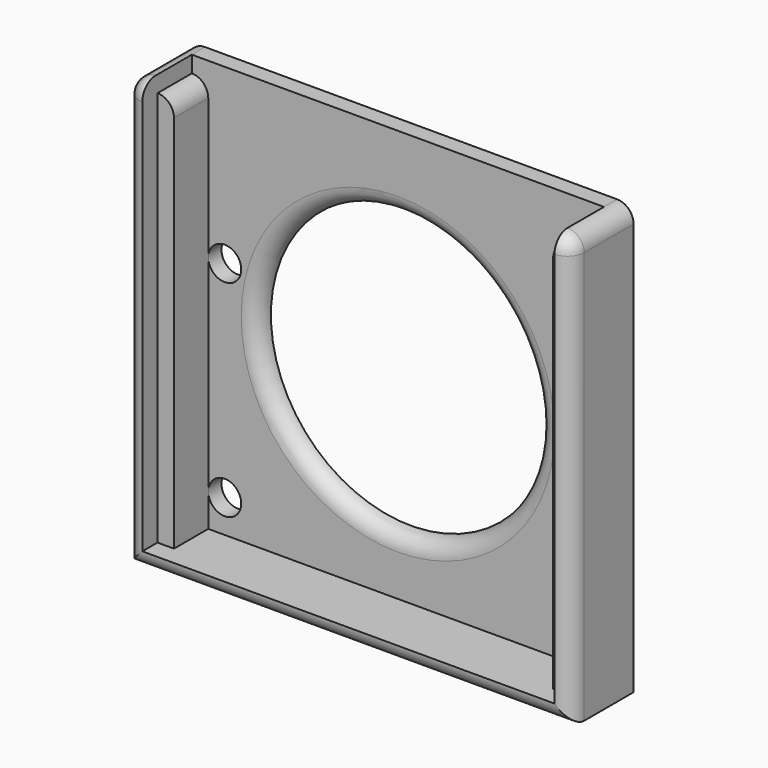
from build123d import *

# Parameters (mm, degrees)
F0_W     = 23
F0_H     = 1
F0_W_2   = 1
F1_DEPTH = 3.75
F2_DEPTH = 2.6
F0_R     = 1
F0_R_2   = 8.5
F3_DEPTH = 1
F4_R     = 0.99999


# Not quite as in the source:
# - a fillet or chamfer is up to 0.001 mm smaller than in the source, because OpenCascade refuses the exact size


with BuildPart() as f1:
    # F0 (on Front) → F1 (new body)
    with BuildSketch(Plane.XZ):
        Polygon((-12.5, -13), (-12.5, -12), (-12.5, 12), (-12.5, 13), (-13.5, 13), (-13.5, -13), align=None)
        Polygon((12.5, 12), (12.5, -12), (12.5, -13), (13.5, -13), (13.5, 13), (12.5, 13), align=None)
        with Locations((0, -12.5)):
            Rectangle(F0_W, F0_H)
        with Locations((-12, -12.5)):
            Rectangle(F0_W_2, F0_H)
        with Locations((12, -12.5)):
            Rectangle(F0_W_2, F0_H)
    extrude(amount=F1_DEPTH)

    # F0 (on Front) → F2 (join)
    with BuildSketch(Plane.XZ):
        Polygon((-12.5, -12), (-11.5, -12), (-11.5, -10), (-11.5, 2.5), (-11.5, 12), (-12.5, 12), align=None)
        Polygon((11.5, -12), (12.5, -12), (12.5, 12), (11.5, 12), (11.5, 2.5), (11.5, -10), align=None)
    extrude(amount=F2_DEPTH)

    # F0 (on Front) → F3 (join)
    with BuildSketch(Plane.XZ):
        Polygon((-11.5, -12), (11.5, -12), (11.5, -10), (11.5, 2.5), (11.5, 12), (-11.5, 12), (-11.5, 2.5), (-11.5, -10), align=None)
        with BuildLine():
            ThreePointArc((-9.5, -10), (-10.5, -11), (-11.5, -10))
            ThreePointArc((-11.5, -10), (-10.5, -9), (-9.5, -10))
        make_face(mode=Mode.SUBTRACT)
        with Locations((10.5, -10)):
            Circle(F0_R, mode=Mode.SUBTRACT)
        with BuildLine():
            ThreePointArc((-9.5, 2.5), (-10.5, 1.5), (-11.5, 2.5))
            ThreePointArc((-11.5, 2.5), (-10.5, 3.5), (-9.5, 2.5))
        make_face(mode=Mode.SUBTRACT)
        Circle(F0_R_2, mode=Mode.SUBTRACT)
        with Locations((10.5, 2.5)):
            Circle(F0_R, mode=Mode.SUBTRACT)
        with Locations((0, 12.5)):
            Rectangle(F0_W, F0_H)
        Polygon((-12.5, -13), (-12.5, -12), (-12.5, 12), (-12.5, 13), (-13.5, 13), (-13.5, -13), align=None)
        Polygon((-12.5, -12), (-11.5, -12), (-11.5, -10), (-11.5, 2.5), (-11.5, 12), (-12.5, 12), align=None)
        with Locations((-12, 12.5)):
            Rectangle(F0_W_2, F0_H)
        with Locations((-12, -12.5)):
            Rectangle(F0_W_2, F0_H)
        with Locations((0, -12.5)):
            Rectangle(F0_W, F0_H)
        with Locations((12, -12.5)):
            Rectangle(F0_W_2, F0_H)
        Polygon((11.5, -12), (12.5, -12), (12.5, 12), (11.5, 12), (11.5, 2.5), (11.5, -10), align=None)
        Polygon((12.5, 12), (12.5, -12), (12.5, -13), (13.5, -13), (13.5, 13), (12.5, 13), align=None)
        with Locations((12, 12.5)):
            Rectangle(F0_W_2, F0_H)
    extrude(amount=-F3_DEPTH)

    # F4 (radius 1 in the source; OpenCascade refuses exactly that, so slightly less here)
    f4_edges = [f1.edges().sort_by_distance(p)[0] for p in [
        (-13.5, -3.75, 0),
        (13.5, -3.75, 0),
        (0, -3.75, -13),
        (-13.5, -1.375, 13),
        (13.5, -1.375, 13),
        (-13, -3.75, 13),
        (13, -3.75, 13),
        (11.5, -1.3, 12),
        (-11.5, -1.3, 12),
        (-8.5, 0, 0),
    ]]
    fillet(f4_edges, radius=F4_R)


solid = f1.part
